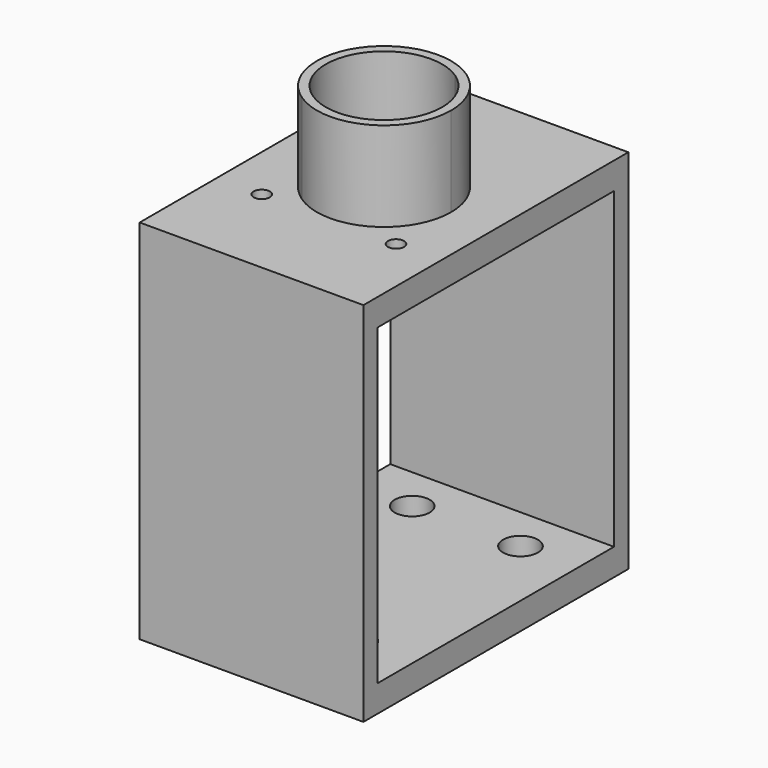
from build123d import *

# Parameters (mm, degrees)
F0_W      = 37
F0_H      = 41
F1_DEPTH  = 25
F2_W      = 33
F2_H      = 35
F3_DEPTH  = 26
F5_DEPTH  = 25
F6_DEPTH  = 10
F7_R      = 1.95
F8_DEPTH  = 4
F9_R      = 0.9
F10_DEPTH = 5


# Not quite as in the source:
# - a feature names something its author has since deleted; it is built from what else it names


with BuildPart() as f1:
    # F0 (on Right) → F1 (new body)
    with BuildSketch(Plane.YZ):
        with Locations((63.15469, -20.5)):
            Rectangle(F0_W, F0_H)
    extrude(amount=F1_DEPTH)

    # F2 (on Right) → F3 (cut)
    with BuildSketch(Plane.YZ):
        with Locations((63.15469, -20.5)):
            Rectangle(F2_W, F2_H)
    extrude(amount=F3_DEPTH, mode=Mode.SUBTRACT)

    # F4 (on Top) → F5 (cut)
    with BuildSketch(Plane.XY):
        with BuildLine():
            ThreePointArc((16.139073, 68.540518), (7.114172, 66.793763), (8.860927, 57.768861))
            Line((8.860927, 57.768861), (16.139073, 68.540518))
        make_face()
        with BuildLine():
            Line((16.139073, 68.540518), (8.860927, 57.768861))
            ThreePointArc((8.860927, 57.768861), (15.549264, 57.414308), (19, 63.15469))
            ThreePointArc((19, 63.15469), (18.240382, 66.203954), (16.139073, 68.540518))
        make_face()
    extrude(amount=-F5_DEPTH, mode=Mode.SUBTRACT)

    # F4 (on Top) → F6 (join)
    with BuildSketch(Plane.XY):
        with BuildLine():
            ThreePointArc((16.698931, 69.369107), (6.285583, 67.35362), (8.301069, 56.940272))
            Line((8.301069, 56.940272), (8.860927, 57.768861))
            ThreePointArc((8.860927, 57.768861), (7.114172, 66.793763), (16.139073, 68.540518))
            Line((16.139073, 68.540518), (16.698931, 69.369107))
        make_face()
        with BuildLine():
            Line((8.860927, 57.768861), (8.301069, 56.940272))
            ThreePointArc((8.301069, 56.940272), (16.018382, 56.531172), (20, 63.15469))
            ThreePointArc((20, 63.15469), (19.123518, 66.673072), (16.698931, 69.369107))
            Line((16.698931, 69.369107), (16.139073, 68.540518))
            ThreePointArc((16.139073, 68.540518), (18.240382, 66.203954), (19, 63.15469))
            ThreePointArc((19, 63.15469), (15.549264, 57.414308), (8.860927, 57.768861))
        make_face()
    extrude(amount=F6_DEPTH)

    # F7 (on face) → F8 (cut)
    with BuildSketch(Plane(origin=(0, 0, -41), x_dir=(1, 0, 0), z_dir=(0, 0, -1))):
        with Locations((6.45, -51.65469)):
            Circle(F7_R)
        with Locations((18.55, -51.65469)):
            Circle(F7_R)
        with Locations((18.55, -74.65469)):
            Circle(F7_R)
        with Locations((6.45, -74.65469)):
            Circle(F7_R)
    extrude(amount=-F8_DEPTH, mode=Mode.SUBTRACT)

    # F9 (on face) → F10 (cut)
    with BuildSketch(Plane.XY):
        with Locations((5, 55.45569)):
            Circle(F9_R)
        with Locations((20, 55.45569)):
            Circle(F9_R)
    extrude(amount=-F10_DEPTH, mode=Mode.SUBTRACT)


solid = f1.part
